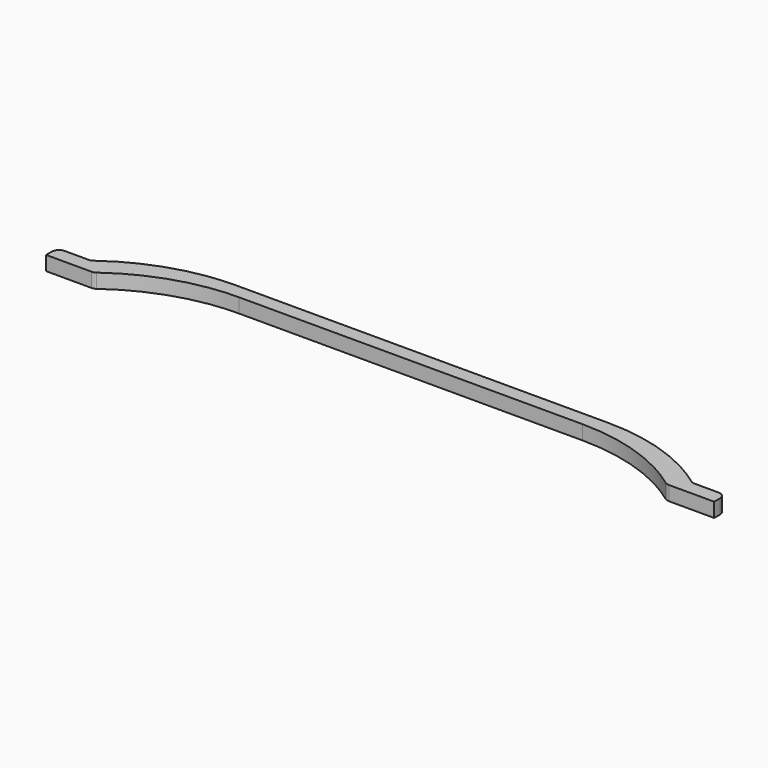
from build123d import *

# Parameters (mm, degrees)
F3_DEPTH = 19.05
F4_R     = 9.525
F5_R     = 254


# Not quite as in the source:
# - a variable given as a bare number and used for a length is read in inches; the dataset says mm whatever the document's units were


with BuildPart() as f3:
    # F2 (on Top) → F3 (new body)
    with BuildSketch(Plane.XY):
        Polygon((0, 19.05), (0, 0), (69.85, 0), (69.85, 50.8), (444.5, 50.8), (819.15, 50.8), (819.15, 0), (889, 0), (889, 19.05), (838.2, 19.05), (838.2, 69.85), (444.5, 69.85), (50.8, 69.85), (50.8, 19.05), align=None)
    extrude(amount=F3_DEPTH)

    # F4
    f4_edges = [f3.edges().sort_by_distance(p)[0] for p in [
        (69.85, 0, 9.525),
        (50.8, 19.05, 9.525),
        (819.15, 0, 9.525),
        (838.2, 19.05, 9.525),
        (0, 19.05, 9.525),
        (889, 19.05, 9.525),
    ]]
    fillet(f4_edges, radius=F4_R)

    # F5
    f5_edges = [f3.edges().sort_by_distance(p)[0] for p in [
        (69.85, 50.8, 9.525),
        (50.8, 69.85, 9.525),
        (819.15, 50.8, 9.525),
        (838.2, 69.85, 9.525),
    ]]
    fillet(f5_edges, radius=F5_R)


solid = f3.part
